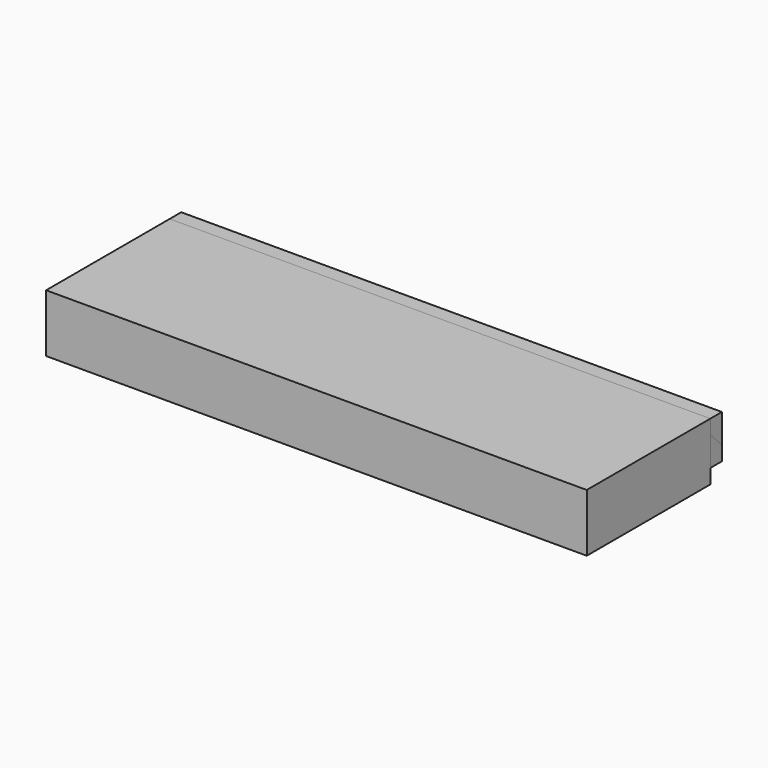
from build123d import *

# Parameters (mm, degrees)
F0_W      = 203.2
F0_H      = 76.2
F1_DEPTH  = 355.6
F3_DEPTH  = 355.6
F6_R      = 3.175
F7_DEPTH  = 57.2937
F6_R_2    = 4.7625
F8_DEPTH  = 6.35
F10_ANGLE = -180


# Not quite as in the source:
# - a feature names something its author has since deleted; it is built from what else it names


with BuildPart() as f1:
    # F0 (on Right) → F1 (new body, symmetric)
    with BuildSketch(Plane.YZ):
        Rectangle(F0_W, F0_H)
    extrude(amount=F1_DEPTH, both=True)


with BuildPart() as f3:
    # F2 (on Right) → F3 (new body, symmetric)
    with BuildSketch(Plane.YZ):
        Polygon((101.6, 19.05), (120.65, 0), (120.65, 38.1), (101.6, 38.1), align=None)
    extrude(amount=F3_DEPTH, both=True)


with BuildPart() as f4_1:
    # F4: copy of F3
    add(f3.part)


with BuildPart() as f4_1_1:
    # F5: moved
    add(f4_1.part.moved(Location((0, 38.2427, -39.84957))))


with BuildPart() as f3_1:
    add(f3.part)

    # F6 (on face) → F7 (cut, through all)
    with BuildSketch(Plane.XZ.offset(-101.6)):
        with Locations((0, 28.575)):
            Circle(F6_R)
        with Locations((-228.6, 28.575)):
            Circle(F6_R)
        with Locations((228.6, 28.575)):
            Circle(F6_R)
    extrude(amount=-F7_DEPTH, mode=Mode.SUBTRACT)

    # F6 (on face) → F8 (cut)
    with BuildSketch(Plane.XZ.offset(-101.6)):
        with Locations((228.6, 28.575)):
            Circle(F6_R_2)
        with Locations((228.6, 28.575)):
            Circle(F6_R, mode=Mode.SUBTRACT)
        with Locations((-228.6, 28.575)):
            Circle(F6_R_2)
        with Locations((-228.6, 28.575)):
            Circle(F6_R, mode=Mode.SUBTRACT)
        with Locations((0, 28.575)):
            Circle(F6_R_2)
        with Locations((0, 28.575)):
            Circle(F6_R, mode=Mode.SUBTRACT)
        with Locations((228.6, 28.575)):
            Circle(F6_R)
        with Locations((0, 28.575)):
            Circle(F6_R)
        with Locations((-228.6, 28.575)):
            Circle(F6_R)
    extrude(amount=-F8_DEPTH, mode=Mode.SUBTRACT)


with BuildPart() as f10_1:
    # F10: copy of F3
    add(f3_1.part.rotate(Axis((0, 101.6, 19.05), (-1, 0, 0)), F10_ANGLE))


with BuildPart() as f10_1_1:
    # F11: moved
    add(f10_1.part.moved(Location((0, 19.05, -19.05))))


solid = Compound([f1.part, f3_1.part, f10_1_1.part])
